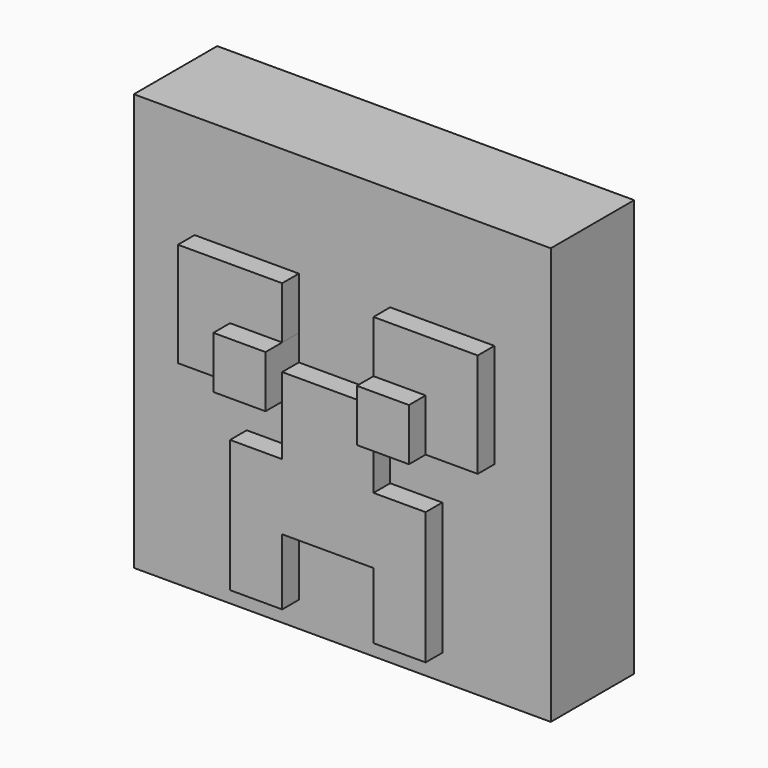
from build123d import *

# Parameters (mm, degrees)
F1_DEPTH = 7.62
F2_DEPTH = 8.89
F3_DEPTH = 7.62
F0_W     = 25.4
F0_H     = 25.4
F4_DEPTH = 6.35


# Not quite as in the source:
# - a feature names something its author has since deleted; it is built from what else it names


with BuildPart() as f1:
    # F0 (on Front) → F1 (new body)
    with BuildSketch(Plane.XZ):
        Polygon((-8.9963801613, 0), (-5.8213801613, 0), (-5.8213801613, 3.1752641518), (-2.6463801613, 3.1752641518), (-2.6463801613, 6.3505283036), (-8.9963801613, 6.3505283036), align=None)
    extrude(amount=F1_DEPTH)


with BuildPart() as f1b:
    # F0 (on Front) → F1, piece 2 (new body)
    with BuildSketch(Plane.XZ):
        Polygon((2.9162198387, 6.3505283036), (2.9162198387, 3.1752641518), (6.0912198387, 3.1752641518), (6.0912198387, 0), (9.2662198387, 0), (9.2662198387, 6.3505283036), align=None)
    extrude(amount=F1_DEPTH)


with BuildPart() as f2:
    # F0 (on Front) → F2 (new body)
    with BuildSketch(Plane.XZ):
        Polygon((-5.8213801613, 0), (-2.6463801613, 0), (-2.6463801613, 1.5876320759), (-2.6463801613, 3.1752641518), (-5.8213801613, 3.1752641518), align=None)
    extrude(amount=F2_DEPTH)


with BuildPart() as f2b:
    # F0 (on Front) → F2, piece 2 (new body)
    with BuildSketch(Plane.XZ):
        Polygon((2.9162198387, 3.1752641518), (2.9162198387, 1.5876320759), (2.9162198387, 0), (6.0912198387, 0), (6.0912198387, 3.1752641518), align=None)
    extrude(amount=F2_DEPTH)


with BuildPart() as f3:
    # F0 (on Front) → F3 (new body)
    with BuildSketch(Plane.XZ):
        Polygon((-2.6463801613, 1.5876320759), (-2.6463801613, 0), (-2.6463801613, -3.0838879648), (-5.8213801613, -3.0838879648), (-5.8213801613, -11.1415497959), (-2.6463801613, -11.1415497959), (-2.6463801613, -7.1127188803), (2.9162198387, -7.1127188803), (2.9162198387, -11.1415497959), (6.0912198387, -11.1415497959), (6.0912198387, -3.0838879648), (2.9162198387, -3.0838879648), (2.9162198387, 0), (2.9162198387, 1.5876320759), align=None)
    extrude(amount=F3_DEPTH)


with BuildPart() as f4:
    # F0 (on Front) → F4 (new body)
    with BuildSketch(Plane.XZ):
        Rectangle(F0_W, F0_H)
        Polygon((-2.6463801613, -3.0838879648), (-2.6463801613, 0), (-5.8213801613, 0), (-8.9963801613, 0), (-8.9963801613, 6.3505283036), (-2.6463801613, 6.3505283036), (-2.6463801613, 3.1752641518), (-2.6463801613, 1.5876320759), (2.9162198387, 1.5876320759), (2.9162198387, 3.1752641518), (2.9162198387, 6.3505283036), (9.2662198387, 6.3505283036), (9.2662198387, 0), (6.0912198387, 0), (2.9162198387, 0), (2.9162198387, -3.0838879648), (6.0912198387, -3.0838879648), (6.0912198387, -11.1415497959), (2.9162198387, -11.1415497959), (2.9162198387, -7.1127188803), (-2.6463801613, -7.1127188803), (-2.6463801613, -11.1415497959), (-5.8213801613, -11.1415497959), (-5.8213801613, -3.0838879648), align=None, mode=Mode.SUBTRACT)
    extrude(amount=F4_DEPTH)


solid = Compound([f1.part, f1b.part, f2.part, f2b.part, f3.part, f4.part])
